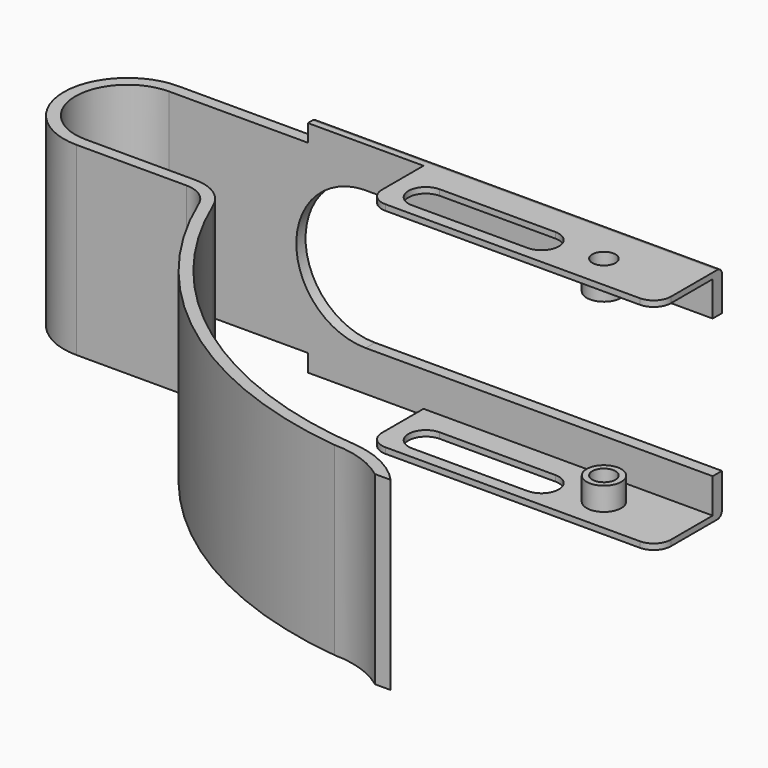
from build123d import *

# Parameters (mm, degrees)
F1_DEPTH  = 16
F2_W      = 70
F2_H      = 3
F3_DEPTH  = 2
F4_W      = 50
F4_H      = 14
F5_DEPTH  = 1
F6_R      = 1
F9_DEPTH  = 2
F11_DEPTH = 1.001
F13_D     = 4
F13_DEPTH = 50
F13_TIP   = 1.2017212381
F14_R     = 3
F14_R_2   = 2
F15_DEPTH = 5
F16_R     = 3
F18_D     = 4
F18_DEPTH = 50
F18_START = 37
F18_TIP   = 1.2017212381


# Not quite as in the source:
# - a pattern or mirror of a feature is missing from the dataset's text; its kind, count and spacing are read off the source's solid
# - a feature names something its author has since deleted; it is built from what else it names


with BuildPart() as f1:
    # F0 (on Top) → F1 (new body)
    with BuildSketch(Plane.XY):
        with BuildLine():
            Line((94, 11), (0, 11))
            ThreePointArc((0, 11), (-11, 0), (0, -11))
            Line((0, -11), (19, -11))
            ThreePointArc((19, -11), (21.7681124643, -11.8361612201), (23.6103896104, -14.064978646))
            ThreePointArc((23.6103896104, -14.064978646), (46.8644288503, -43.8489365308), (81.9993431207, -57.7547729841))
            ThreePointArc((81.9993431207, -57.7547729841), (87.0632727772, -58.5972193444), (91.5997631119, -61))
            Line((91.5997631119, -61), (94.3248553538, -61))
            ThreePointArc((94.3248553538, -61), (89.9506080698, -57.6601123846), (84.7034264019, -56))
            ThreePointArc((84.7034264019, -56), (49.0672193413, -42.9854179344), (25.4545454545, -13.2909701044))
            ThreePointArc((25.4545454545, -13.2909701044), (22.87535745, -10.1706257081), (19, -9))
            Line((19, -9), (0, -9))
            ThreePointArc((0, -9), (-9, 0), (0, 9))
            Line((0, 9), (94, 9))
            Line((94, 9), (94, 11))
        make_face()
    extrude(amount=F1_DEPTH)

    # F2 (on face) → F3 (join)
    with BuildSketch(Plane(origin=(0, 11, 0), x_dir=(-1, 0, 0), z_dir=(0, 1, 0))):
        with Locations((-59, 17.5)):
            Rectangle(F2_W, F2_H)
    extrude(amount=-F3_DEPTH)

    # F4 (on face) → F5 (join)
    with BuildSketch(Plane.XY.offset(19)):
        with Locations((69, 4)):
            Rectangle(F4_W, F4_H)
    extrude(amount=-F5_DEPTH)

    # F6
    f6_edges = [f1.edges().sort_by_distance(p)[0] for p in [
        (59, 11, 19),
    ]]
    fillet(f6_edges, radius=F6_R)

    # F7: F1 across face


with BuildPart() as f1_1:
    add(f1.part)
    add(f1.part.mirror(Plane(origin=(39.0198924269, -12.8147332924, 0), x_dir=(1, 0, 0), z_dir=(0, 0, -1))))

    # F8 (on face) → F9 (cut)
    with BuildSketch(Plane(origin=(0, 11, 0), x_dir=(-1, 0, 0), z_dir=(0, 1, 0))):
        with BuildLine():
            Line((-94, -12), (-34, -12))
            ThreePointArc((-34, -12), (-22.001130085, -0.1646838272), (-33.6706633635, 11.9954798728))
            Line((-33.6706633635, 11.9954798728), (-34.3293366365, 11.9954798728))
            Line((-34.3293366365, 11.9954798728), (-94, 11.9954798728))
            Line((-94, 11.9954798728), (-94, -12))
        make_face()
    extrude(amount=-F9_DEPTH, mode=Mode.SUBTRACT)

    # F10 (on face) → F11 (cut, through all)
    with BuildSketch(Plane(origin=(0, 0, 18), x_dir=(1, 0, 0), z_dir=(0, 0, -1))):
        with BuildLine():
            ThreePointArc((50, 1), (47, -2), (50, -5))
            Line((50, -5), (70, -5))
            ThreePointArc((70, -5), (73, -2), (70, 1))
            Line((70, 1), (50, 1))
        make_face()
    f11 = extrude(amount=-F11_DEPTH, mode=Mode.SUBTRACT)

    # F11_copies: F11 across plane
    add(f11.mirror(Plane(origin=(0, 0, 0), x_dir=(-1, 0, 0), z_dir=(0, 0, -1))), mode=Mode.SUBTRACT)

    # F13 (one way)
    with BuildSketch(Plane(origin=(0, 0, 18), x_dir=(1, 0, 0), z_dir=(0, 0, -1))):
        with Locations((80, -3)):
            Circle(F13_D / 2)
    extrude(amount=-F13_DEPTH, mode=Mode.SUBTRACT)
    with Locations(Plane(origin=(0, 0, 18), x_dir=(1, 0, 0), z_dir=(0, 0, -1))):
        with Locations((80, -3)):
            with Locations((0, 0, -(F13_DEPTH + F13_TIP / 2))):  # 118° drill point
                Cone(0, F13_D / 2, F13_TIP, mode=Mode.SUBTRACT)

    # F14 (on face) → F15 (join)
    with BuildSketch(Plane.XY.offset(19)):
        with Locations((80, 3)):
            Circle(F14_R)
        with Locations((80, 3)):
            Circle(F14_R_2, mode=Mode.SUBTRACT)
    f15 = extrude(amount=-F15_DEPTH)

    # F15_copies: F15 across plane
    add(f15.mirror(Plane(origin=(0, 0, 0), x_dir=(-1, 0, 0), z_dir=(0, 0, -1))))

    # F16
    f16_edges = [f1_1.edges().sort_by_distance(p)[0] for p in [
        (94, -3, 18.5),
        (44, -3, 18.5),
        (44, -3, -18.5),
        (94, -3, -18.5),
    ]]
    fillet(f16_edges, radius=F16_R)

    # F18
    # its depths count from where the whole tool has entered the part; down to there all is cleared
    with Locations(Plane.XY.offset(19).offset(-F18_START)):
        with Locations((79.9801871181, 3.0164394993)):
            Hole(F18_D / 2, depth=F18_DEPTH)
            with Locations((0, 0, -(F18_DEPTH + F18_TIP / 2))):  # 118° drill point
                Cone(0, F18_D / 2, F18_TIP, mode=Mode.SUBTRACT)


solid = f1_1.part
